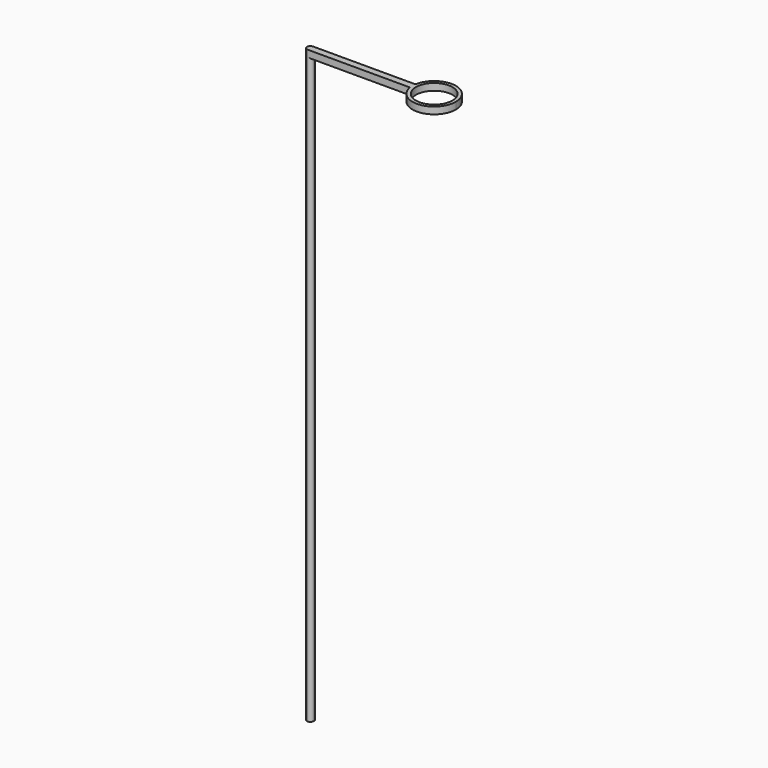
from build123d import *

# Parameters (mm, degrees)
F0_R     = 3.175
F1_DEPTH = 1.190625
F2_DEPTH = 101.6


# Not quite as in the source:
# - a length typed as a fraction of an inch, garbled in the dataset ("3 / 203.2 mm" for 3/8 in), is restored


with BuildPart() as f1:
    # F0 (on Top) → F1 (new body)
    with BuildSketch(Plane.XY):
        with BuildLine():
            ThreePointArc((-3.7230175094, -0.5953125), (-3.7703125, 0), (-3.7230175094, 0.5953125))
            Line((-3.7230175094, 0.5953125), (-21.5030175094, 0.5953125))
            ThreePointArc((-21.5030175094, 0.5953125), (-21.0820680037, 0.4209495057), (-20.9077050094, 0))
            ThreePointArc((-20.9077050094, 0), (-21.0820680037, -0.4209495057), (-21.5030175094, -0.5953125))
            Line((-21.5030175094, -0.5953125), (-3.7230175094, -0.5953125))
        make_face()
        with BuildLine():
            ThreePointArc((-3.7230175094, -0.5953125), (0.2985941178, -3.7584701543), (3.7703125, 0))
            ThreePointArc((3.7703125, 0), (0.2985941178, 3.7584701543), (-3.7230175094, 0.5953125))
            ThreePointArc((-3.7230175094, 0.5953125), (-3.7703125, 0), (-3.7230175094, -0.5953125))
        make_face()
        Circle(F0_R, mode=Mode.SUBTRACT)
        with BuildLine():
            ThreePointArc((-20.9077050094, 0), (-21.0820680037, 0.4209495057), (-21.5030175094, 0.5953125))
            ThreePointArc((-21.5030175094, 0.5953125), (-22.0983300094, 0), (-21.5030175094, -0.5953125))
            ThreePointArc((-21.5030175094, -0.5953125), (-21.0820680037, -0.4209495057), (-20.9077050094, 0))
        make_face()
    extrude(amount=F1_DEPTH)

    # F0 (on Top) → F2 (join)
    with BuildSketch(Plane.XY):
        with BuildLine():
            ThreePointArc((-20.9077050094, 0), (-21.0820680037, 0.4209495057), (-21.5030175094, 0.5953125))
            ThreePointArc((-21.5030175094, 0.5953125), (-22.0983300094, 0), (-21.5030175094, -0.5953125))
            ThreePointArc((-21.5030175094, -0.5953125), (-21.0820680037, -0.4209495057), (-20.9077050094, 0))
        make_face()
    extrude(amount=-F2_DEPTH)


solid = f1.part
